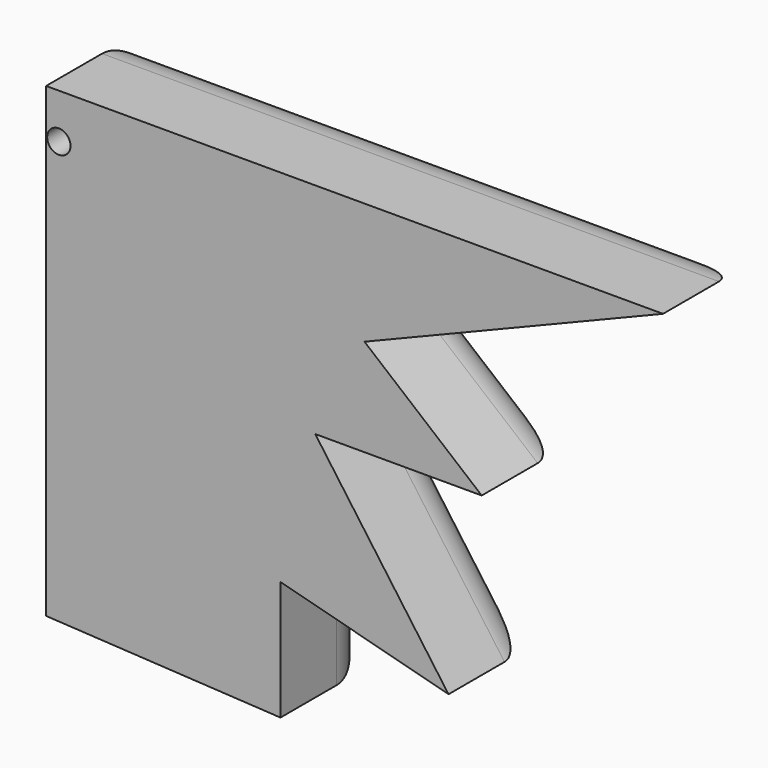
from build123d import *

# Parameters (mm, degrees)
F1_DEPTH     = 25
F2_R         = 2.5
F3_DEPTH     = 46.9
F4_T1_DEPTH  = 150
F4_T3_DEPTH  = 182.2274848408
F4_T5_DEPTH  = 100.3173754326
F4_T10_DEPTH = 75.5924176596
F4_T15_DEPTH = 87.245278787
F4_T20_DEPTH = 99.0010747165
F4_T25_DEPTH = 85.6788355908
F4_T30_DEPTH = 82.646426835
F4_T35_DEPTH = 119.0871070802
F4_T41_DEPTH = 75.5924176596
F4_T45_DEPTH = 87.245278787
F4_T52_DEPTH = 85.6788355908
F4_T56_DEPTH = 99.0010747165
F4_T63_DEPTH = 119.0871070802
F4_T67_DEPTH = 82.646426835


# Not quite as in the source:
# - a fillet or chamfer that OpenCascade refuses, or shapes differently, is made with other operations: its cross-section is extruded or revolved along the edge and cut away or added


with BuildPart() as f1:
    # F0 (on Front) → F1 (new body)
    with BuildSketch(Plane.XZ):
        Polygon((49.0980417262, 68.0754659733), (-83.1294431146, 68.0754659733), (-83.1294431146, -31.9245340267), (-32.8924826343, -34.7681359889), (-32.8924826343, -9.1757183293), (3.1264783981, -18.6543911301), (-25.4433550304, 21.1560339021), (10.2354805604, 21.1560339021), (-14.8830008989, 42.00911699), align=None)
    extrude(amount=F1_DEPTH)

    # F2 (on Front) → F3 (cut)
    with BuildSketch(Plane.XZ):
        with Locations((-80.3935006261, 58.4694631398)):
            Circle(F2_R)
    extrude(amount=F3_DEPTH, mode=Mode.SUBTRACT)

    # F4: fillet of radius 10 on 9 edges, made by hand

    # F4_s2 → F4_t1 (cut)
    with BuildSketch(Plane.XY.offset(-56.9245340267)):
        with BuildLine():
            ThreePointArc((-83.1294431146, -10), (-80.2005109264, -2.9289321881), (-73.1294431146, 0))
            Line((-73.1294431146, 0), (-83.1294431146, 0))
            Line((-83.1294431146, 0), (-83.1294431146, -10))
        make_face()
    extrude(amount=F4_T1_DEPTH, mode=Mode.SUBTRACT)

    # F4_s4 → F4_t3 (cut)
    with BuildSketch(Plane.YZ.offset(-108.1294431146)):
        with BuildLine():
            ThreePointArc((-10, 68.0754659733), (-2.9289321881, 65.1465337851), (0, 58.0754659733))
            Line((0, 58.0754659733), (0, 68.0754659733))
            Line((0, 68.0754659733), (-10, 68.0754659733))
        make_face()
    extrude(amount=F4_T3_DEPTH, mode=Mode.SUBTRACT)

    # F4_s6 → F4_t5 (cut)
    with BuildSketch(Plane(origin=(-106.0227160465, 0, 6.0012867121), x_dir=(0, 1, 0), z_dir=(0.9984018453, 0, -0.0565133205))):
        with BuildLine():
            ThreePointArc((0, -26.5714345391), (-2.9289321881, -33.6425023509), (-10, -36.5714345391))
            Line((-10, -36.5714345391), (0, -36.5714345391))
            Line((0, -36.5714345391), (0, -26.5714345391))
        make_face()
    extrude(amount=F4_T5_DEPTH, mode=Mode.SUBTRACT)


with BuildPart() as f4_tool8:
    # F4_s9 → F4_t10 (new body)
    with BuildSketch(Plane.XY.offset(-59.7681359889)):
        with BuildLine():
            ThreePointArc((-42.8924826343, 0), (-35.8214148224, -2.9289321881), (-32.8924826343, -10))
            Line((-32.8924826343, -10), (-32.8924826343, 0))
            Line((-32.8924826343, 0), (-42.8924826343, 0))
        make_face()
    extrude(amount=F4_T10_DEPTH)

    split(bisect_by=Plane(origin=(-4.3886140602, 0, -16.676735461), x_dir=(0, 1, 0), z_dir=(-0.2544932703, 0, -0.9670745449)), keep=Keep.TOP)


with BuildPart() as f1_1:
    add(f1.part)

    # F4_t7: cut F4_tool8
    add(f4_tool8.part, mode=Mode.SUBTRACT)


with BuildPart() as f4_tool13:
    # F4_s14 → F4_t15 (new body)
    with BuildSketch(Plane(origin=(-52.6807321964, 0, 13.8633488887), x_dir=(0, 1, 0), z_dir=(0.9670745449, 0, -0.2544932703))):
        with BuildLine():
            ThreePointArc((0, -7.2445191005), (-2.9289321881, -14.3155869123), (-10, -17.2445191005))
            Line((-10, -17.2445191005), (0, -17.2445191005))
            Line((0, -17.2445191005), (0, -7.2445191005))
        make_face()
    extrude(amount=F4_T15_DEPTH)

    split(bisect_by=Plane.YZ.offset(-32.8924826343), keep=Keep.TOP)


with BuildPart() as f1_2:
    add(f1_1.part)

    # F4_t12: cut F4_tool13
    add(f4_tool13.part, mode=Mode.SUBTRACT)


with BuildPart() as f4_tool18:
    # F4_s19 → F4_t20 (new body)
    with BuildSketch(Plane(origin=(24.4753258646, 0, -34.1049634717), x_dir=(0, 1, 0), z_dir=(-0.5830450371, 0, 0.8124398345))):
        with BuildLine():
            ThreePointArc((0, 18.3362745772), (-2.9289321881, 11.2652067653), (-10, 8.3362745772))
            Line((-10, 8.3362745772), (0, 8.3362745772))
            Line((0, 8.3362745772), (0, 18.3362745772))
        make_face()
    extrude(amount=F4_T20_DEPTH)

    split(bisect_by=Plane.XY.offset(21.1560339021), keep=Keep.BOTTOM)


with BuildPart() as f1_3:
    add(f1_2.part)

    # F4_t17: cut F4_tool18
    add(f4_tool18.part, mode=Mode.SUBTRACT)


with BuildPart() as f4_tool23:
    # F4_s24 → F4_t25 (new body)
    with BuildSketch(Plane.YZ.offset(-50.4433550304)):
        with BuildLine():
            ThreePointArc((0, 31.1560339021), (-2.9289321881, 24.0849660902), (-10, 21.1560339021))
            Line((-10, 21.1560339021), (0, 21.1560339021))
            Line((0, 21.1560339021), (0, 31.1560339021))
        make_face()
    extrude(amount=F4_T25_DEPTH)

    split(bisect_by=Plane(origin=(-6.7727215377, 0, -4.8604235206), x_dir=(0, 1, 0), z_dir=(0.8124398345, 0, 0.5830450371)), keep=Keep.TOP)


with BuildPart() as f1_4:
    add(f1_3.part)

    # F4_t22: cut F4_tool23
    add(f4_tool23.part, mode=Mode.SUBTRACT)


with BuildPart() as f4_tool28:
    # F4_s29 → F4_t30 (new body)
    with BuildSketch(Plane(origin=(14.897118547, 0, -12.3674216268), x_dir=(0, 1, 0), z_dir=(-0.769409822, 0, 0.6387554507))):
        with BuildLine():
            ThreePointArc((0, -12.8156292772), (-2.9289321881, -19.8866970891), (-10, -22.8156292772))
            Line((-10, -22.8156292772), (0, -22.8156292772))
            Line((0, -22.8156292772), (0, -12.8156292772))
        make_face()
    extrude(amount=F4_T30_DEPTH)

    split(bisect_by=Plane(origin=(-16.7971177223, 0, 41.2292916688), x_dir=(0, 1, 0), z_dir=(0.377296866, 0, -0.9260923684)), keep=Keep.TOP)


with BuildPart() as f1_5:
    add(f1_4.part)

    # F4_t27: cut F4_tool28
    add(f4_tool28.part, mode=Mode.SUBTRACT)


with BuildPart() as f4_tool33:
    # F4_s34 → F4_t35 (new body)
    with BuildSketch(Plane(origin=(-21.2381923878, 0, -8.6525963291), x_dir=(0, 1, 0), z_dir=(0.9260923684, 0, 0.377296866))):
        with BuildLine():
            ThreePointArc((-10, 44.5196322457), (-2.9289321881, 47.4485644338), (0, 54.5196322457))
            Line((0, 54.5196322457), (0, 44.5196322457))
            Line((0, 44.5196322457), (-10, 44.5196322457))
        make_face()
    extrude(amount=F4_T35_DEPTH)

    split(bisect_by=Plane(origin=(14.5736075628, 0, 17.5545692605), x_dir=(0, 1, 0), z_dir=(0.6387554507, 0, 0.769409822)), keep=Keep.TOP)


with BuildPart() as f1_6:
    add(f1_5.part)

    # F4_t32: cut F4_tool33
    add(f4_tool33.part, mode=Mode.SUBTRACT)


with BuildPart() as f4_tool39:
    # F4_s40 → F4_t41 (new body)
    with BuildSketch(Plane.XY.offset(-59.7681359889)):
        with BuildLine():
            ThreePointArc((-42.8924826343, 0), (-35.8214148224, -2.9289321881), (-32.8924826343, -10))
            Line((-32.8924826343, -10), (-32.8924826343, 0))
            Line((-32.8924826343, 0), (-42.8924826343, 0))
        make_face()
    extrude(amount=F4_T41_DEPTH)

    split(bisect_by=Plane(origin=(-4.3886140602, 0, -16.676735461), x_dir=(0, 1, 0), z_dir=(0.2544932703, 0, 0.9670745449)), keep=Keep.TOP)


with BuildPart() as f4_tool43:
    # F4_s44 → F4_t45 (new body)
    with BuildSketch(Plane(origin=(-52.6807321964, 0, 13.8633488887), x_dir=(0, 1, 0), z_dir=(0.9670745449, 0, -0.2544932703))):
        with BuildLine():
            ThreePointArc((0, -7.2445191005), (-2.9289321881, -14.3155869123), (-10, -17.2445191005))
            Line((-10, -17.2445191005), (0, -17.2445191005))
            Line((0, -17.2445191005), (0, -7.2445191005))
        make_face()
    extrude(amount=F4_T45_DEPTH)

    split(bisect_by=Plane.YZ.offset(-32.8924826343), keep=Keep.BOTTOM)


with BuildPart() as f4_tool39_1:
    add(f4_tool39.part)

    # F4_t47: intersect F4_tool43
    add(f4_tool43.part, mode=Mode.INTERSECT)


with BuildPart() as f1_7:
    add(f1_6.part)

    # F4_t37: cut F4_tool39
    add(f4_tool39_1.part, mode=Mode.SUBTRACT)


with BuildPart() as f4_tool50:
    # F4_s51 → F4_t52 (new body)
    with BuildSketch(Plane.YZ.offset(-50.4433550304)):
        with BuildLine():
            ThreePointArc((0, 31.1560339021), (-2.9289321881, 24.0849660902), (-10, 21.1560339021))
            Line((-10, 21.1560339021), (0, 21.1560339021))
            Line((0, 21.1560339021), (0, 31.1560339021))
        make_face()
    extrude(amount=F4_T52_DEPTH)

    split(bisect_by=Plane(origin=(-6.7727215377, 0, -4.8604235206), x_dir=(0, 1, 0), z_dir=(-0.8124398345, 0, -0.5830450371)), keep=Keep.TOP)


with BuildPart() as f4_tool54:
    # F4_s55 → F4_t56 (new body)
    with BuildSketch(Plane(origin=(24.4753258646, 0, -34.1049634717), x_dir=(0, 1, 0), z_dir=(-0.5830450371, 0, 0.8124398345))):
        with BuildLine():
            ThreePointArc((0, 18.3362745772), (-2.9289321881, 11.2652067653), (-10, 8.3362745772))
            Line((-10, 8.3362745772), (0, 8.3362745772))
            Line((0, 8.3362745772), (0, 18.3362745772))
        make_face()
    extrude(amount=F4_T56_DEPTH)

    split(bisect_by=Plane.XY.offset(21.1560339021), keep=Keep.TOP)


with BuildPart() as f4_tool50_1:
    add(f4_tool50.part)

    # F4_t58: intersect F4_tool54
    add(f4_tool54.part, mode=Mode.INTERSECT)


with BuildPart() as f1_8:
    add(f1_7.part)

    # F4_t48: cut F4_tool50
    add(f4_tool50_1.part, mode=Mode.SUBTRACT)


with BuildPart() as f4_tool61:
    # F4_s62 → F4_t63 (new body)
    with BuildSketch(Plane(origin=(-21.2381923878, 0, -8.6525963291), x_dir=(0, 1, 0), z_dir=(0.9260923684, 0, 0.377296866))):
        with BuildLine():
            ThreePointArc((-10, 44.5196322457), (-2.9289321881, 47.4485644338), (0, 54.5196322457))
            Line((0, 54.5196322457), (0, 44.5196322457))
            Line((0, 44.5196322457), (-10, 44.5196322457))
        make_face()
    extrude(amount=F4_T63_DEPTH)

    split(bisect_by=Plane(origin=(14.5736075628, 0, 17.5545692605), x_dir=(0, 1, 0), z_dir=(-0.6387554507, 0, -0.769409822)), keep=Keep.TOP)


with BuildPart() as f4_tool65:
    # F4_s66 → F4_t67 (new body)
    with BuildSketch(Plane(origin=(14.897118547, 0, -12.3674216268), x_dir=(0, 1, 0), z_dir=(-0.769409822, 0, 0.6387554507))):
        with BuildLine():
            ThreePointArc((0, -12.8156292772), (-2.9289321881, -19.8866970891), (-10, -22.8156292772))
            Line((-10, -22.8156292772), (0, -22.8156292772))
            Line((0, -22.8156292772), (0, -12.8156292772))
        make_face()
    extrude(amount=F4_T67_DEPTH)

    split(bisect_by=Plane(origin=(-16.7971177223, 0, 41.2292916688), x_dir=(0, 1, 0), z_dir=(-0.377296866, 0, 0.9260923684)), keep=Keep.TOP)


with BuildPart() as f4_tool61_1:
    add(f4_tool61.part)

    # F4_t69: intersect F4_tool65
    add(f4_tool65.part, mode=Mode.INTERSECT)


with BuildPart() as f1_9:
    add(f1_8.part)

    # F4_t59: cut F4_tool61
    add(f4_tool61_1.part, mode=Mode.SUBTRACT)


solid = f1_9.part
